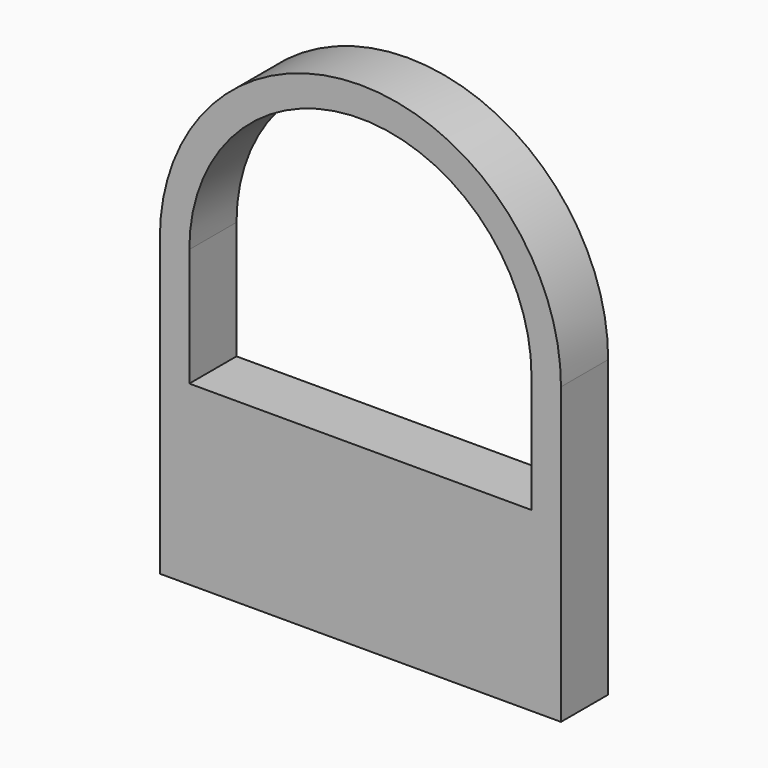
from build123d import *

# Parameters (mm, degrees)
F1_DEPTH = 6.35


# Not quite as in the source:
# - ends of sketch curves that miss each other by under 0.0002 mm in the source are joined


with BuildPart() as f1:
    # F0 (on Front) → F1 (new body, symmetric)
    with BuildSketch(Plane.XZ):
        Polygon((-36.8300005794, 19.05), (-43.18, 19.05), (-43.18, -19.05), (43.18, -19.05), (43.18, 19.05), (36.8300005794, 19.05), align=None)
        with BuildLine():
            Line((-43.18, 44.45), (-43.18, 19.05))
            Line((-43.18, 19.05), (-36.8300005794, 19.05))
            Line((-36.8300005794, 19.05), (-36.8300005794, 44.45))
            ThreePointArc((-36.8300005794, 44.45), (0, 81.28), (36.83, 44.45))
            Line((36.83, 44.45), (36.8300005794, 19.05))
            Line((36.8300005794, 19.05), (43.18, 19.05))
            Line((43.18, 19.05), (43.18, 44.45))
            ThreePointArc((43.18, 44.45), (0, 87.63), (-43.18, 44.45))
        make_face()
    extrude(amount=F1_DEPTH, both=True)


solid = f1.part
